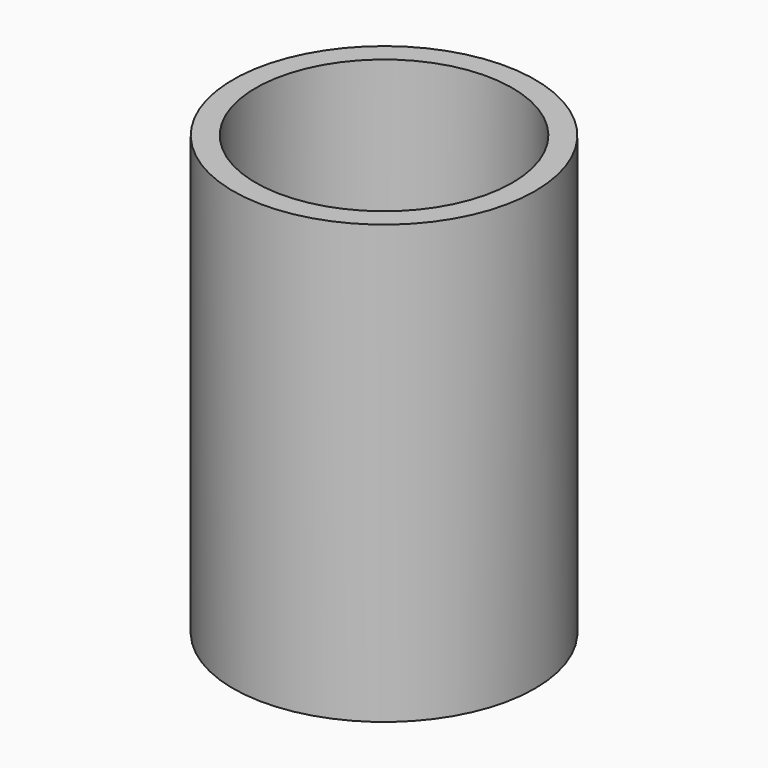
from build123d import *

# Parameters (mm, degrees)
F0_R     = 12.7
F0_R_2   = 10.795
F1_DEPTH = 33.02
F2_R     = 12.7
F2_R_2   = 10.795
F3_DEPTH = 3.81


with BuildPart() as f1:
    # F0 (on Top) → F1 (new body)
    with BuildSketch(Plane.XY):
        Circle(F0_R)
        Circle(F0_R_2, mode=Mode.SUBTRACT)
    extrude(amount=F1_DEPTH)

    # F2 (on face) → F3 (join)
    with BuildSketch(Plane(origin=(0, 0, 0), x_dir=(1, 0, 0), z_dir=(0, 0, -1))):
        Circle(F2_R)
        Circle(F2_R_2, mode=Mode.SUBTRACT)
        Circle(F2_R_2)
    extrude(amount=F3_DEPTH)


solid = f1.part
